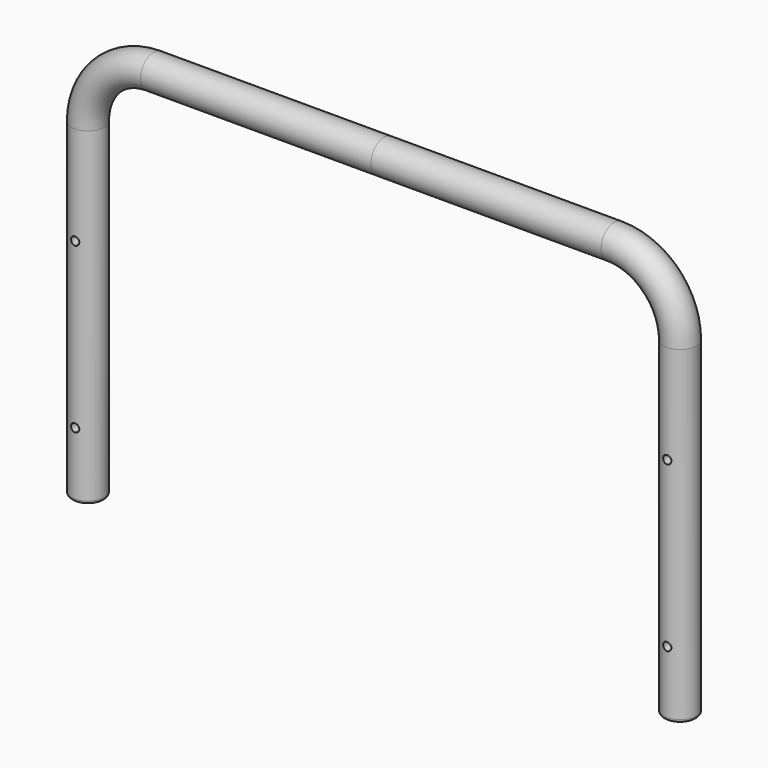
from build123d import *

# Parameters (mm, degrees)
F0_R          = 12.7
F4_R          = 3.175
F5_DEPTH      = 25.4
F5_DEPTH_BACK = 25.4
F6_R          = 2.54


with BuildPart() as f2:
    # F2: sweep along a path in F1
    with BuildLine(Plane.XZ) as f2_path:
        Line((0, 304.8), (-177.8, 304.8))
        ThreePointArc((-177.8, 304.8), (-213.7210244843, 289.9210244843), (-228.6, 254))
        Line((-228.6, 254), (-228.6, 0))
    # F0 (on Top) → F2 (sweep)
    with BuildSketch(Plane.XY):
        with Locations((-228.6, 0)):
            Circle(F0_R)
    sweep(path=f2_path.line)

    # F3: F2 across plane


with BuildPart() as f2_1:
    add(f2.part)
    add(f2.part.mirror(Plane.YZ))

    # F4 (on Front) → F5 (cut, two sides)
    with BuildSketch(Plane.XZ) as f5_sk:
        with BuildLine():
            ThreePointArc((-228.6, 53.975), (-231.775, 50.8), (-228.6, 47.625))
            Line((-228.6, 47.625), (-228.6, 50.8))
            Line((-228.6, 50.8), (-228.6, 53.975))
        make_face()
        with BuildLine():
            ThreePointArc((-225.425, 177.8), (-230.8450640303, 180.0450640303), (-228.6, 174.625))
            ThreePointArc((-228.6, 174.625), (-226.3549359697, 175.5549359697), (-225.425, 177.8))
        make_face()
        with BuildLine():
            Line((-228.6, 50.8), (-228.6, 47.625))
            ThreePointArc((-228.6, 47.625), (-226.3549359697, 48.5549359697), (-225.425, 50.8))
            ThreePointArc((-225.425, 50.8), (-226.3549359697, 53.0450640303), (-228.6, 53.975))
            Line((-228.6, 53.975), (-228.6, 50.8))
        make_face()
        with Locations((228.6, 177.8)):
            Circle(F4_R)
        with Locations((228.6, 50.8)):
            Circle(F4_R)
    extrude(amount=F5_DEPTH, mode=Mode.SUBTRACT)
    extrude(f5_sk.sketch, amount=-F5_DEPTH_BACK, mode=Mode.SUBTRACT)

    # F6
    f6_edges = [f2_1.edges().sort_by_distance(p)[0] for p in [
        (241.3, 0, 0),
        (-241.3, 0, 0),
    ]]
    fillet(f6_edges, radius=F6_R)


solid = f2_1.part
